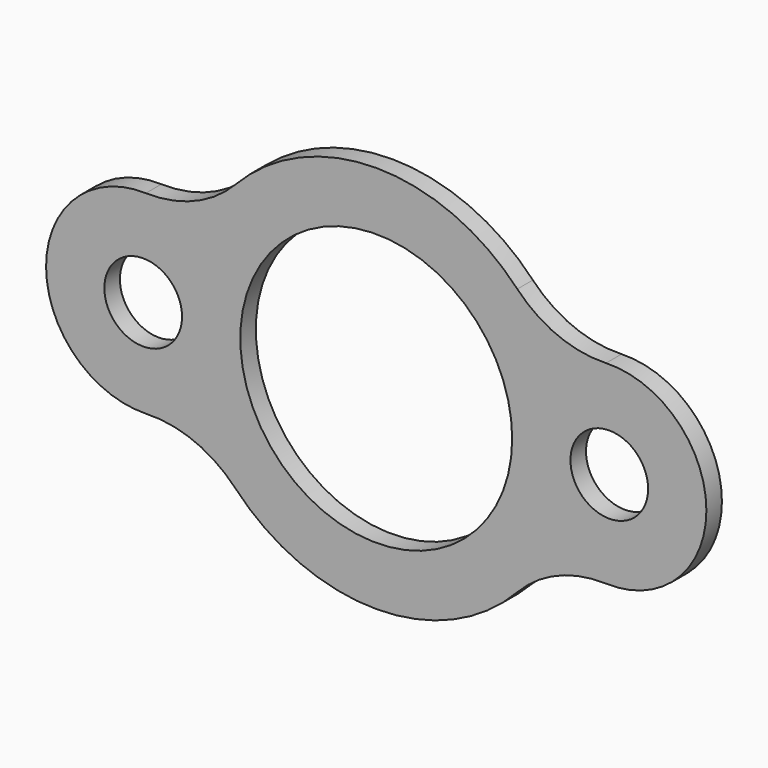
from build123d import *

# Parameters (mm, degrees)
F0_R     = 12.7
F0_R_2   = 44.45
F1_DEPTH = 6.35


# Not quite as in the source:
# - a length typed as a fraction of an inch, garbled in the dataset ("3 / 203.2 mm" for 3/8 in), is restored


with BuildPart() as f1:
    # F0 (on Front) → F1 (new body)
    with BuildSketch(Plane.XZ):
        with BuildLine():
            ThreePointArc((-75.1176136364, -31.7315448688), (-59.3475236203, -34.5646316236), (-46.13671875, -43.6308741946))
            ThreePointArc((-46.13671875, -43.6308741946), (0, -63.5), (46.13671875, -43.6308741946))
            ThreePointArc((46.13671875, -43.6308741946), (59.3475236203, -34.5646316236), (75.1176136364, -31.7315448688))
            ThreePointArc((75.1176136364, -31.7315448688), (107.95, 0), (75.1176136364, 31.7315448688))
            ThreePointArc((75.1176136364, 31.7315448688), (59.3475236203, 34.5646316236), (46.13671875, 43.6308741946))
            ThreePointArc((46.13671875, 43.6308741946), (0.1332471885, 63.4998601982), (-45.9532044665, 43.8241143579))
            ThreePointArc((-45.9532044665, 43.8241143579), (-59.3485408179, 34.6632102418), (-75.3109250125, 31.7375494591))
            ThreePointArc((-75.3109250125, 31.7375494591), (-107.9498527345, -0.0967023051), (-75.1176136364, -31.7315448688))
        make_face()
        with Locations((-76.2, 0)):
            Circle(F0_R, mode=Mode.SUBTRACT)
        Circle(F0_R_2, mode=Mode.SUBTRACT)
        with Locations((76.2, 0)):
            Circle(F0_R, mode=Mode.SUBTRACT)
    extrude(amount=F1_DEPTH)


solid = f1.part
